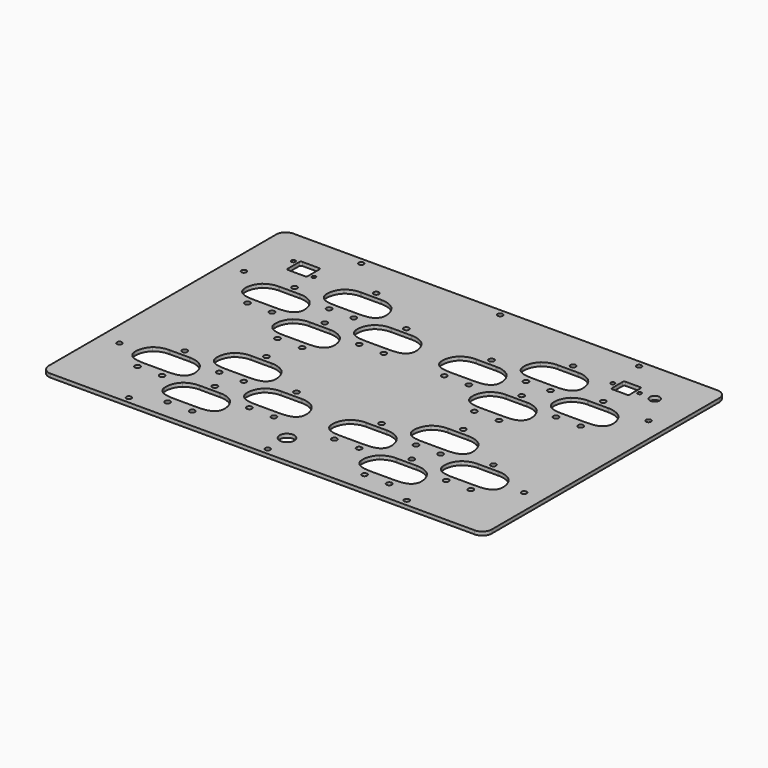
from build123d import *

# Parameters (mm, degrees)
F0_R     = 2.1
F0_R_2   = 2.2
F0_R_3   = 6
F0_R_4   = 1.625
F0_R_5   = 1.6
F0_R_6   = 4.05
F1_DEPTH = 3


# Not quite as in the source:
# - the dataset's text gives a spline's control points without its knots; the knots are read off the source's solid


with BuildPart() as f1:
    # F0 (on Top) → F1 (new body)
    with BuildSketch(Plane.XY):
        with BuildLine():
            Line((174.5, 124.8), (-174.5, 124.8))
            ThreePointArc((-174.5, 124.8), (-180.0154328933, 122.5154328933), (-182.3, 117))
            Line((-182.3, 117), (-182.3, -117))
            ThreePointArc((-182.3, -117), (-180.0154328933, -122.5154328933), (-174.5, -124.8))
            Line((-174.5, -124.8), (174.5, -124.8))
            ThreePointArc((174.5, -124.8), (180.0154328933, -122.5154328933), (182.3, -117))
            Line((182.3, -117), (182.3, 117))
            ThreePointArc((182.3, 117), (180.0154328933, 122.5154328933), (174.5, 124.8))
        make_face()
        with Locations((-114.33, -119.5)):
            Circle(F0_R, mode=Mode.SUBTRACT)
        with Locations((-137.12, -82.102)):
            Circle(F0_R_2, mode=Mode.SUBTRACT)
        with Locations((-166.5, -64)):
            Circle(F0_R, mode=Mode.SUBTRACT)
        with Locations((-116.88, -82.102)):
            Circle(F0_R_2, mode=Mode.SUBTRACT)
        with BuildLine():
            Line((-135.6612948233, -51.451130735), (-135.115026498, -51.4620000001))
            Line((-135.115026498, -51.4620000001), (-118.8944121234, -51.4620000001))
            Line((-118.8944121234, -51.4620000001), (-118.3330315352, -51.4511211146))
            ThreePointArc((-118.3330315352, -51.4511211146), (-112.5954929046, -52.4136608229), (-107.487280821, -55.1979024679))
            ThreePointArc((-107.487280821, -55.1979024679), (-103.7289593809, -60.9649156398), (-102.7756384695, -67.7821438311))
            add(Edge.make_bspline(
                [(-102.7756384695, -67.7821438311), (-102.8317808557, -68.4791518436), (-103.1342622315, -69.8522558093), (-104.1227442667, -71.7376713061), (-105.3617732771, -73.0712234734), (-106.5853971676, -73.93803931), (-107.9464485907, -74.6539246569), (-109.8851336202, -75.2963766675), (-112.5588382079, -75.7473994177), (-115.5566427484, -75.9552688032), (-117.7556974045, -75.97825395), (-118.9009345935, -75.9720000001)],
                knots=[0, 0, 0, 0, 0.125, 0.25, 0.375, 0.4375, 0.5, 0.625, 0.75, 0.875, 0.9999501857, 0.9999501857, 0.9999501857, 0.9999501857], degree=3))
            Line((-118.9009345935, -75.9720000001), (-135.1072635354, -75.9720000001))
            Line((-135.1072635354, -75.9720000001), (-135.1086333173, -75.9720000001))
            add(Edge.make_bspline(
                [(-151.2339294072, -67.7821438309), (-151.177741554, -68.4797163167), (-150.8726831114, -69.8530561961), (-149.8774581613, -71.7367332364), (-148.6340002387, -73.0683891085), (-147.4094063644, -73.9344572306), (-146.0489657757, -74.6503376548), (-144.1131861346, -75.2935631846), (-141.4445788782, -75.7458922174), (-138.4515011772, -75.954911071), (-136.2539205452, -75.9782540848), (-135.1086333173, -75.9720000001)],
                knots=[0, 0, 0, 0, 0.125, 0.25, 0.375, 0.4375, 0.5, 0.625, 0.75, 0.875, 0.9999501867, 0.9999501867, 0.9999501867, 0.9999501867], degree=3))
            ThreePointArc((-151.2339294072, -67.7821438309), (-150.2806084958, -60.9649156397), (-146.5222870557, -55.1979024678))
            ThreePointArc((-146.5222870557, -55.1979024678), (-141.4068713777, -52.411174013), (-135.6612948233, -51.451130735))
        make_face(mode=Mode.SUBTRACT)
        with Locations((-91.12, -108.602)):
            Circle(F0_R_2, mode=Mode.SUBTRACT)
        with Locations((-70.88, -108.602)):
            Circle(F0_R_2, mode=Mode.SUBTRACT)
        with BuildLine():
            Line((-89.6612948233, -77.951130735), (-89.115026498, -77.9620000001))
            Line((-89.115026498, -77.9620000001), (-72.8944121234, -77.9620000001))
            Line((-72.8944121234, -77.9620000001), (-72.3330315352, -77.9511211146))
            ThreePointArc((-72.3330315352, -77.9511211146), (-66.5954929046, -78.9136608229), (-61.487280821, -81.6979024679))
            ThreePointArc((-61.487280821, -81.6979024679), (-57.7289593809, -87.4649156398), (-56.7756384695, -94.2821438311))
            add(Edge.make_bspline(
                [(-56.7756384695, -94.2821438311), (-56.8318288861, -94.9783630519), (-57.1341419789, -96.3506841544), (-58.1219861034, -98.2355446893), (-59.3608225377, -99.5692757568), (-60.5843212484, -100.4362682741), (-61.9452692843, -101.1523501476), (-63.8838615244, -101.7950820951), (-66.5575009571, -102.2464909201), (-69.5556737218, -102.4548208566), (-71.7552033004, -102.4781051534), (-72.9009345935, -102.4720000001)],
                knots=[0.0001387542, 0.0001387542, 0.0001387542, 0.0001387542, 0.125, 0.25, 0.375, 0.4375, 0.5, 0.625, 0.75, 0.875, 1, 1, 1, 1], degree=3))
            Line((-72.9009345935, -102.4720000001), (-89.1072635354, -102.4720000001))
            Line((-89.1072635354, -102.4720000001), (-89.1086333173, -102.4720000001))
            add(Edge.make_bspline(
                [(-105.2339294072, -94.2821438309), (-105.177741554, -94.9797163167), (-104.8726831114, -96.3530561961), (-103.8774581613, -98.2367332364), (-102.6340002387, -99.5683891085), (-101.4094063644, -100.4344572306), (-100.0489657757, -101.1503376548), (-98.1131861346, -101.7935631846), (-95.4445788782, -102.2458922174), (-92.4515011772, -102.454911071), (-90.2539205452, -102.4782540848), (-89.1086333173, -102.4720000001)],
                knots=[0, 0, 0, 0, 0.125, 0.25, 0.375, 0.4375, 0.5, 0.625, 0.75, 0.875, 0.9999501867, 0.9999501867, 0.9999501867, 0.9999501867], degree=3))
            ThreePointArc((-105.2339294072, -94.2821438309), (-104.2806084958, -87.4649156397), (-100.5222870557, -81.6979024678))
            ThreePointArc((-100.5222870557, -81.6979024678), (-95.4068713777, -78.911174013), (-89.6612948233, -77.951130735))
        make_face(mode=Mode.SUBTRACT)
        with Locations((-81, -72.692)):
            Circle(F0_R_2, mode=Mode.SUBTRACT)
        with Locations((-45.12, -82.102)):
            Circle(F0_R_2, mode=Mode.SUBTRACT)
        with Locations((-24.88, -82.102)):
            Circle(F0_R_2, mode=Mode.SUBTRACT)
        with BuildLine():
            Line((-43.6612948233, -51.451130735), (-43.115026498, -51.4620000001))
            Line((-43.115026498, -51.4620000001), (-26.8944121234, -51.4620000001))
            Line((-26.8944121234, -51.4620000001), (-26.3330315352, -51.4511211146))
            ThreePointArc((-26.3330315352, -51.4511211146), (-20.5954929046, -52.4136608229), (-15.487280821, -55.1979024679))
            ThreePointArc((-15.487280821, -55.1979024679), (-11.7289593809, -60.9649156398), (-10.7756384695, -67.7821438311))
            add(Edge.make_bspline(
                [(-10.7756384695, -67.7821438311), (-10.8317808557, -68.4791518436), (-11.1342622315, -69.8522558093), (-12.1227442667, -71.7376713061), (-13.3617732771, -73.0712234734), (-14.5853971676, -73.93803931), (-15.9464485907, -74.6539246569), (-17.8851336202, -75.2963766675), (-20.5588382079, -75.7473994177), (-23.5566427484, -75.9552688032), (-25.7556974045, -75.97825395), (-26.9009345935, -75.9720000001)],
                knots=[0, 0, 0, 0, 0.125, 0.25, 0.375, 0.4375, 0.5, 0.625, 0.75, 0.875, 0.9999501857, 0.9999501857, 0.9999501857, 0.9999501857], degree=3))
            Line((-26.9009345935, -75.9720000001), (-43.1072635354, -75.9720000001))
            Line((-43.1072635354, -75.9720000001), (-43.1086333173, -75.9720000001))
            add(Edge.make_bspline(
                [(-59.2339294072, -67.7821438309), (-59.177741554, -68.4797163167), (-58.8726831114, -69.8530561961), (-57.8774581613, -71.7367332364), (-56.6340002387, -73.0683891085), (-55.4094063644, -73.9344572306), (-54.0489657757, -74.6503376548), (-52.1131861346, -75.2935631846), (-49.4445788782, -75.7458922174), (-46.4515011772, -75.954911071), (-44.2539205452, -75.9782540848), (-43.1086333173, -75.9720000001)],
                knots=[0, 0, 0, 0, 0.125, 0.25, 0.375, 0.4375, 0.5, 0.625, 0.75, 0.875, 0.9999501867, 0.9999501867, 0.9999501867, 0.9999501867], degree=3))
            ThreePointArc((-59.2339294072, -67.7821438309), (-58.2806084958, -60.9649156397), (-54.5222870557, -55.1979024678))
            ThreePointArc((-54.5222870557, -55.1979024678), (-49.4068713777, -52.411174013), (-43.6612948233, -51.451130735))
        make_face(mode=Mode.SUBTRACT)
        with Locations((-127, -46.192)):
            Circle(F0_R_2, mode=Mode.SUBTRACT)
        with Locations((-91.12, -55.602)):
            Circle(F0_R_2, mode=Mode.SUBTRACT)
        with Locations((-70.88, -55.602)):
            Circle(F0_R_2, mode=Mode.SUBTRACT)
        with BuildLine():
            Line((-89.6612948233, -24.951130735), (-89.115026498, -24.9620000001))
            Line((-89.115026498, -24.9620000001), (-72.8944121234, -24.9620000001))
            Line((-72.8944121234, -24.9620000001), (-72.3330315352, -24.9511211146))
            ThreePointArc((-72.3330315352, -24.9511211146), (-66.5954929046, -25.9136608229), (-61.487280821, -28.6979024679))
            ThreePointArc((-61.487280821, -28.6979024679), (-57.7289593809, -34.4649156398), (-56.7756384695, -41.2821438311))
            add(Edge.make_bspline(
                [(-56.7756384695, -41.2821438311), (-56.8317808557, -41.9791518436), (-57.1342622315, -43.3522558093), (-58.1227442667, -45.2376713061), (-59.3617732771, -46.5712234734), (-60.5853971676, -47.43803931), (-61.9464485907, -48.1539246569), (-63.8851336202, -48.7963766675), (-66.5588382079, -49.2473994177), (-69.5566427484, -49.4552688032), (-71.7556974045, -49.47825395), (-72.9009345935, -49.4720000001)],
                knots=[0, 0, 0, 0, 0.125, 0.25, 0.375, 0.4375, 0.5, 0.625, 0.75, 0.875, 0.9999501857, 0.9999501857, 0.9999501857, 0.9999501857], degree=3))
            Line((-72.9009345935, -49.4720000001), (-89.1072635354, -49.4720000001))
            Line((-89.1072635354, -49.4720000001), (-89.1086333173, -49.4720000001))
            add(Edge.make_bspline(
                [(-105.2339294072, -41.2821438309), (-105.177741554, -41.9797163167), (-104.8726831114, -43.3530561961), (-103.8774581613, -45.2367332364), (-102.6340002387, -46.5683891085), (-101.4094063644, -47.4344572306), (-100.0489657757, -48.1503376548), (-98.1131861346, -48.7935631846), (-95.4445788782, -49.2458922174), (-92.4515011772, -49.454911071), (-90.2539205452, -49.4782540848), (-89.1086333173, -49.4720000001)],
                knots=[0, 0, 0, 0, 0.125, 0.25, 0.375, 0.4375, 0.5, 0.625, 0.75, 0.875, 0.9999501867, 0.9999501867, 0.9999501867, 0.9999501867], degree=3))
            ThreePointArc((-105.2339294072, -41.2821438309), (-104.2806084958, -34.4649156397), (-100.5222870557, -28.6979024678))
            ThreePointArc((-100.5222870557, -28.6979024678), (-95.4068713777, -25.911174013), (-89.6612948233, -24.951130735))
        make_face(mode=Mode.SUBTRACT)
        with Locations((-35, -46.192)):
            Circle(F0_R_2, mode=Mode.SUBTRACT)
        with Locations((-81, -19.692)):
            Circle(F0_R_2, mode=Mode.SUBTRACT)
        with Locations((0, -119.5)):
            Circle(F0_R, mode=Mode.SUBTRACT)
        with Locations((0, -99.8)):
            Circle(F0_R_3, mode=Mode.SUBTRACT)
        with Locations((70.88, -108.602)):
            Circle(F0_R_2, mode=Mode.SUBTRACT)
        with Locations((91.12, -108.602)):
            Circle(F0_R_2, mode=Mode.SUBTRACT)
        with Locations((24.88, -82.102)):
            Circle(F0_R_2, mode=Mode.SUBTRACT)
        with Locations((45.12, -82.102)):
            Circle(F0_R_2, mode=Mode.SUBTRACT)
        with BuildLine():
            Line((26.3387051767, -51.451130735), (26.884973502, -51.4620000001))
            Line((26.884973502, -51.4620000001), (43.1055878766, -51.4620000001))
            Line((43.1055878766, -51.4620000001), (43.6669684648, -51.4511211146))
            ThreePointArc((43.6669684648, -51.4511211146), (49.4045070954, -52.4136608229), (54.512719179, -55.1979024679))
            ThreePointArc((54.512719179, -55.1979024679), (58.2710406191, -60.9649156398), (59.2243615305, -67.7821438311))
            add(Edge.make_bspline(
                [(59.2243615305, -67.7821438311), (59.1682191443, -68.4791518436), (58.8657377685, -69.8522558093), (57.8772557333, -71.7376713061), (56.6382267229, -73.0712234734), (55.4146028324, -73.93803931), (54.0535514093, -74.6539246569), (52.1148663798, -75.2963766675), (49.4411617921, -75.7473994177), (46.4433572516, -75.9552688032), (44.2443025955, -75.97825395), (43.0990654065, -75.9720000001)],
                knots=[0, 0, 0, 0, 0.125, 0.25, 0.375, 0.4375, 0.5, 0.625, 0.75, 0.875, 0.9999501857, 0.9999501857, 0.9999501857, 0.9999501857], degree=3))
            Line((43.0990654065, -75.9720000001), (26.8927364646, -75.9720000001))
            Line((26.8927364646, -75.9720000001), (26.8913666827, -75.9720000001))
            add(Edge.make_bspline(
                [(10.7660705928, -67.7821438309), (10.822258446, -68.4797163167), (11.1273168886, -69.8530561961), (12.1225418387, -71.7367332364), (13.3659997613, -73.0683891085), (14.5905936356, -73.9344572306), (15.9510342243, -74.6503376548), (17.8868138654, -75.2935631846), (20.5554211218, -75.7458922174), (23.5484988228, -75.954911071), (25.7460794548, -75.9782540848), (26.8913666827, -75.9720000001)],
                knots=[0, 0, 0, 0, 0.125, 0.25, 0.375, 0.4375, 0.5, 0.625, 0.75, 0.875, 0.9999501867, 0.9999501867, 0.9999501867, 0.9999501867], degree=3))
            ThreePointArc((10.7660705928, -67.7821438309), (11.7193915042, -60.9649156397), (15.4777129443, -55.1979024678))
            ThreePointArc((15.4777129443, -55.1979024678), (20.5931286223, -52.411174013), (26.3387051767, -51.451130735))
        make_face(mode=Mode.SUBTRACT)
        with BuildLine():
            Line((72.3387051767, -77.951130735), (72.884973502, -77.9620000001))
            Line((72.884973502, -77.9620000001), (89.1055878766, -77.9620000001))
            Line((89.1055878766, -77.9620000001), (89.6669684648, -77.9511211146))
            ThreePointArc((89.6669684648, -77.9511211146), (95.4045070954, -78.9136608229), (100.512719179, -81.6979024679))
            ThreePointArc((100.512719179, -81.6979024679), (104.2710406191, -87.4649156398), (105.2243615305, -94.2821438311))
            add(Edge.make_bspline(
                [(105.2243615305, -94.2821438311), (105.1682191443, -94.9791518436), (104.8657377685, -96.3522558093), (103.8772557333, -98.2376713061), (102.6382267229, -99.5712234734), (101.4146028324, -100.43803931), (100.0535514093, -101.1539246569), (98.1148663798, -101.7963766675), (95.4411617921, -102.2473994177), (92.4433572516, -102.4552688032), (90.2443025955, -102.47825395), (89.0990654065, -102.4720000001)],
                knots=[0, 0, 0, 0, 0.125, 0.25, 0.375, 0.4375, 0.5, 0.625, 0.75, 0.875, 0.9999501857, 0.9999501857, 0.9999501857, 0.9999501857], degree=3))
            Line((89.0990654065, -102.4720000001), (72.8927364646, -102.4720000001))
            Line((72.8927364646, -102.4720000001), (72.8913666827, -102.4720000001))
            add(Edge.make_bspline(
                [(56.7660705928, -94.2821438309), (56.822258446, -94.9797163167), (57.1273168886, -96.3530561961), (58.1225418387, -98.2367332364), (59.3659997613, -99.5683891085), (60.5905936356, -100.4344572306), (61.9510342243, -101.1503376548), (63.8868138654, -101.7935631846), (66.5554211218, -102.2458922174), (69.5484988228, -102.454911071), (71.7460794548, -102.4782540848), (72.8913666827, -102.4720000001)],
                knots=[0, 0, 0, 0, 0.125, 0.25, 0.375, 0.4375, 0.5, 0.625, 0.75, 0.875, 0.9999501867, 0.9999501867, 0.9999501867, 0.9999501867], degree=3))
            ThreePointArc((56.7660705928, -94.2821438309), (57.7193915042, -87.4649156397), (61.4777129443, -81.6979024678))
            ThreePointArc((61.4777129443, -81.6979024678), (66.5931286223, -78.911174013), (72.3387051767, -77.951130735))
        make_face(mode=Mode.SUBTRACT)
        with Locations((81, -72.692)):
            Circle(F0_R_2, mode=Mode.SUBTRACT)
        with Locations((114.33, -119.5)):
            Circle(F0_R, mode=Mode.SUBTRACT)
        with Locations((116.88, -82.102)):
            Circle(F0_R_2, mode=Mode.SUBTRACT)
        with BuildLine():
            Line((118.3387051767, -51.451130735), (118.884973502, -51.4620000001))
            Line((118.884973502, -51.4620000001), (135.1055878766, -51.4620000001))
            Line((135.1055878766, -51.4620000001), (135.6669684648, -51.4511211146))
            ThreePointArc((135.6669684648, -51.4511211146), (141.4045070954, -52.4136608229), (146.512719179, -55.1979024679))
            ThreePointArc((146.512719179, -55.1979024679), (150.2710406191, -60.9649156398), (151.2243615305, -67.7821438311))
            add(Edge.make_bspline(
                [(151.2243615305, -67.7821438311), (151.1682191443, -68.4791518436), (150.8657377685, -69.8522558093), (149.8772557333, -71.7376713061), (148.6382267229, -73.0712234734), (147.4146028324, -73.93803931), (146.0535514093, -74.6539246569), (144.1148663798, -75.2963766675), (141.4411617921, -75.7473994177), (138.4433572516, -75.9552688032), (136.2443025955, -75.97825395), (135.0990654065, -75.9720000001)],
                knots=[0, 0, 0, 0, 0.125, 0.25, 0.375, 0.4375, 0.5, 0.625, 0.75, 0.875, 0.9999501857, 0.9999501857, 0.9999501857, 0.9999501857], degree=3))
            Line((135.0990654065, -75.9720000001), (118.8927364646, -75.9720000001))
            Line((118.8927364646, -75.9720000001), (118.8913666827, -75.9720000001))
            add(Edge.make_bspline(
                [(102.7660705928, -67.7821438309), (102.822258446, -68.4797163167), (103.1273168886, -69.8530561961), (104.1225418387, -71.7367332364), (105.3659997613, -73.0683891085), (106.5905936356, -73.9344572306), (107.9510342243, -74.6503376548), (109.8868138654, -75.2935631846), (112.5554211218, -75.7458922174), (115.5484988228, -75.954911071), (117.7460794548, -75.9782540848), (118.8913666827, -75.9720000001)],
                knots=[0, 0, 0, 0, 0.125, 0.25, 0.375, 0.4375, 0.5, 0.625, 0.75, 0.875, 0.9999501867, 0.9999501867, 0.9999501867, 0.9999501867], degree=3))
            ThreePointArc((102.7660705928, -67.7821438309), (103.7193915042, -60.9649156397), (107.4777129443, -55.1979024678))
            ThreePointArc((107.4777129443, -55.1979024678), (112.5931286223, -52.411174013), (118.3387051767, -51.451130735))
        make_face(mode=Mode.SUBTRACT)
        with Locations((137.12, -82.102)):
            Circle(F0_R_2, mode=Mode.SUBTRACT)
        with Locations((166.5, -64)):
            Circle(F0_R, mode=Mode.SUBTRACT)
        with Locations((35, -46.192)):
            Circle(F0_R_2, mode=Mode.SUBTRACT)
        with Locations((70.88, -55.602)):
            Circle(F0_R_2, mode=Mode.SUBTRACT)
        with Locations((91.12, -55.602)):
            Circle(F0_R_2, mode=Mode.SUBTRACT)
        with BuildLine():
            Line((72.3387051767, -24.951130735), (72.884973502, -24.9620000001))
            Line((72.884973502, -24.9620000001), (89.1055878766, -24.9620000001))
            Line((89.1055878766, -24.9620000001), (89.6669684648, -24.9511211146))
            ThreePointArc((89.6669684648, -24.9511211146), (95.4045070954, -25.9136608229), (100.512719179, -28.6979024679))
            ThreePointArc((100.512719179, -28.6979024679), (104.2710406191, -34.4649156398), (105.2243615305, -41.2821438311))
            add(Edge.make_bspline(
                [(105.2243615305, -41.2821438311), (105.1682191443, -41.9791518436), (104.8657377685, -43.3522558093), (103.8772557333, -45.2376713061), (102.6382267229, -46.5712234734), (101.4146028324, -47.43803931), (100.0535514093, -48.1539246569), (98.1148663798, -48.7963766675), (95.4411617921, -49.2473994177), (92.4433572516, -49.4552688032), (90.2443025955, -49.47825395), (89.0990654065, -49.4720000001)],
                knots=[0, 0, 0, 0, 0.125, 0.25, 0.375, 0.4375, 0.5, 0.625, 0.75, 0.875, 0.9999501857, 0.9999501857, 0.9999501857, 0.9999501857], degree=3))
            Line((89.0990654065, -49.4720000001), (72.8927364646, -49.4720000001))
            Line((72.8927364646, -49.4720000001), (72.8913666827, -49.4720000001))
            add(Edge.make_bspline(
                [(56.7660705928, -41.2821438309), (56.822258446, -41.9797163167), (57.1273168886, -43.3530561961), (58.1225418387, -45.2367332364), (59.3659997613, -46.5683891085), (60.5905936356, -47.4344572306), (61.9510342243, -48.1503376548), (63.8868138654, -48.7935631846), (66.5554211218, -49.2458922174), (69.5484988228, -49.454911071), (71.7460794548, -49.4782540848), (72.8913666827, -49.4720000001)],
                knots=[0, 0, 0, 0, 0.125, 0.25, 0.375, 0.4375, 0.5, 0.625, 0.75, 0.875, 0.9999501867, 0.9999501867, 0.9999501867, 0.9999501867], degree=3))
            ThreePointArc((56.7660705928, -41.2821438309), (57.7193915042, -34.4649156397), (61.4777129443, -28.6979024678))
            ThreePointArc((61.4777129443, -28.6979024678), (66.5931286223, -25.911174013), (72.3387051767, -24.951130735))
        make_face(mode=Mode.SUBTRACT)
        with Locations((81, -19.692)):
            Circle(F0_R_2, mode=Mode.SUBTRACT)
        with Locations((127, -46.192)):
            Circle(F0_R_2, mode=Mode.SUBTRACT)
        with Locations((-137.12, 30.898)):
            Circle(F0_R_2, mode=Mode.SUBTRACT)
        with Locations((-116.88, 30.898)):
            Circle(F0_R_2, mode=Mode.SUBTRACT)
        with BuildLine():
            Line((-135.6612948233, 61.548869265), (-135.115026498, 61.5379999999))
            Line((-135.115026498, 61.5379999999), (-118.8944121234, 61.5379999999))
            Line((-118.8944121234, 61.5379999999), (-118.3330315352, 61.5488788854))
            ThreePointArc((-118.3330315352, 61.5488788854), (-112.5954929046, 60.5863391771), (-107.487280821, 57.8020975321))
            ThreePointArc((-107.487280821, 57.8020975321), (-103.7289593809, 52.0350843602), (-102.7756384695, 45.2178561689))
            add(Edge.make_bspline(
                [(-102.7756384695, 45.2178561689), (-102.8317808557, 44.5208481564), (-103.1342622315, 43.1477441907), (-104.1227442667, 41.2623286939), (-105.3617732771, 39.9287765266), (-106.5853971676, 39.06196069), (-107.9464485907, 38.3460753431), (-109.8851336202, 37.7036233325), (-112.5588382079, 37.2526005823), (-115.5566427484, 37.0447311968), (-117.7556974045, 37.02174605), (-118.9009345935, 37.0279999999)],
                knots=[0, 0, 0, 0, 0.125, 0.25, 0.375, 0.4375, 0.5, 0.625, 0.75, 0.875, 0.9999501857, 0.9999501857, 0.9999501857, 0.9999501857], degree=3))
            Line((-118.9009345935, 37.0279999999), (-135.1072635354, 37.0279999999))
            Line((-135.1072635354, 37.0279999999), (-135.1086333173, 37.0279999999))
            add(Edge.make_bspline(
                [(-151.2339294072, 45.2178561691), (-151.177741554, 44.5202836833), (-150.8726831114, 43.1469438039), (-149.8774581613, 41.2632667636), (-148.6340002387, 39.9316108915), (-147.4094063644, 39.0655427694), (-146.0489657757, 38.3496623452), (-144.1131861346, 37.7064368154), (-141.4445788782, 37.2541077826), (-138.4515011772, 37.045088929), (-136.2539205452, 37.0217459152), (-135.1086333173, 37.0279999999)],
                knots=[0, 0, 0, 0, 0.125, 0.25, 0.375, 0.4375, 0.5, 0.625, 0.75, 0.875, 0.9999501867, 0.9999501867, 0.9999501867, 0.9999501867], degree=3))
            ThreePointArc((-151.2339294072, 45.2178561691), (-150.2806084958, 52.0350843603), (-146.5222870557, 57.8020975322))
            ThreePointArc((-146.5222870557, 57.8020975322), (-141.4068713777, 60.588825987), (-135.6612948233, 61.548869265))
        make_face(mode=Mode.SUBTRACT)
        with Locations((-91.12, 4.398)):
            Circle(F0_R_2, mode=Mode.SUBTRACT)
        with Locations((-70.88, 4.398)):
            Circle(F0_R_2, mode=Mode.SUBTRACT)
        with BuildLine():
            Line((-89.6612948233, 35.048869265), (-89.115026498, 35.0379999999))
            Line((-89.115026498, 35.0379999999), (-72.8944121234, 35.0379999999))
            Line((-72.8944121234, 35.0379999999), (-72.3330315352, 35.0488788854))
            ThreePointArc((-72.3330315352, 35.0488788854), (-66.5954929046, 34.0863391771), (-61.487280821, 31.3020975321))
            ThreePointArc((-61.487280821, 31.3020975321), (-57.7289593809, 25.5350843602), (-56.7756384695, 18.7178561689))
            add(Edge.make_bspline(
                [(-56.7756384695, 18.7178561689), (-56.8317808557, 18.0208481564), (-57.1342622315, 16.6477441907), (-58.1227442667, 14.7623286939), (-59.3617732771, 13.4287765266), (-60.5853971676, 12.56196069), (-61.9464485907, 11.8460753431), (-63.8851336202, 11.2036233325), (-66.5588382079, 10.7526005823), (-69.5566427484, 10.5447311968), (-71.7556974045, 10.52174605), (-72.9009345935, 10.5279999999)],
                knots=[0, 0, 0, 0, 0.125, 0.25, 0.375, 0.4375, 0.5, 0.625, 0.75, 0.875, 0.9999501857, 0.9999501857, 0.9999501857, 0.9999501857], degree=3))
            Line((-72.9009345935, 10.5279999999), (-89.1072635354, 10.5279999999))
            Line((-89.1072635354, 10.5279999999), (-89.1086333173, 10.5279999999))
            add(Edge.make_bspline(
                [(-105.2339294072, 18.7178561691), (-105.177741554, 18.0202836833), (-104.8726831114, 16.6469438039), (-103.8774581613, 14.7632667636), (-102.6340002387, 13.4316108915), (-101.4094063644, 12.5655427694), (-100.0489657757, 11.8496623452), (-98.1131861346, 11.2064368154), (-95.4445788782, 10.7541077826), (-92.4515011772, 10.545088929), (-90.2539205452, 10.5217459152), (-89.1086333173, 10.5279999999)],
                knots=[0, 0, 0, 0, 0.125, 0.25, 0.375, 0.4375, 0.5, 0.625, 0.75, 0.875, 0.9999501867, 0.9999501867, 0.9999501867, 0.9999501867], degree=3))
            ThreePointArc((-105.2339294072, 18.7178561691), (-104.2806084958, 25.5350843603), (-100.5222870557, 31.3020975322))
            ThreePointArc((-100.5222870557, 31.3020975322), (-95.4068713777, 34.088825987), (-89.6612948233, 35.048869265))
        make_face(mode=Mode.SUBTRACT)
        with Locations((-45.12, 30.898)):
            Circle(F0_R_2, mode=Mode.SUBTRACT)
        with Locations((-24.88, 30.898)):
            Circle(F0_R_2, mode=Mode.SUBTRACT)
        with Locations((-81, 40.308)):
            Circle(F0_R_2, mode=Mode.SUBTRACT)
        with Locations((-91.12, 57.398)):
            Circle(F0_R_2, mode=Mode.SUBTRACT)
        with Locations((-70.88, 57.398)):
            Circle(F0_R_2, mode=Mode.SUBTRACT)
        with BuildLine():
            Line((-43.6612948233, 61.548869265), (-43.115026498, 61.5379999999))
            Line((-43.115026498, 61.5379999999), (-26.8944121234, 61.5379999999))
            Line((-26.8944121234, 61.5379999999), (-26.3330315352, 61.5488788854))
            ThreePointArc((-26.3330315352, 61.5488788854), (-20.5954929046, 60.5863391771), (-15.487280821, 57.8020975321))
            ThreePointArc((-15.487280821, 57.8020975321), (-11.7282191214, 52.0352577574), (-10.7742686876, 45.2178561689))
            add(Edge.make_bspline(
                [(-10.7742686876, 45.2178561689), (-10.8304110738, 44.5208481564), (-11.1328924496, 43.1477441907), (-12.1213744847, 41.2623286939), (-13.3604034952, 39.9287765266), (-14.5840273857, 39.06196069), (-15.9450788087, 38.3460753431), (-17.8837638383, 37.7036233325), (-20.557468426, 37.2526005823), (-23.5552729664, 37.0447311968), (-25.7543276226, 37.02174605), (-26.8995648116, 37.0279999999)],
                knots=[0, 0, 0, 0, 0.125, 0.25, 0.375, 0.4375, 0.5, 0.625, 0.75, 0.875, 0.9999501857, 0.9999501857, 0.9999501857, 0.9999501857], degree=3))
            Line((-26.8995648116, 37.0279999999), (-43.1072635354, 37.0279999999))
            add(Edge.make_bspline(
                [(-59.2325596253, 45.2178561691), (-59.1763212388, 44.5210734563), (-58.8714315071, 43.1485163208), (-57.876846428, 41.2653920745), (-56.633580812, 39.9335566586), (-55.4091120122, 39.0673117119), (-54.0487748122, 38.3512348451), (-52.1130880742, 37.7077297918), (-49.4445461628, 37.255015412), (-46.4511010398, 37.0455365283), (-44.2530455057, 37.0218945801), (-43.1072635354, 37.0279999999)],
                knots=[0.0001386451, 0.0001386451, 0.0001386451, 0.0001386451, 0.125, 0.25, 0.375, 0.4375, 0.5, 0.625, 0.75, 0.875, 1, 1, 1, 1], degree=3))
            ThreePointArc((-59.2325596253, 45.2178561691), (-58.2798682404, 52.0349109767), (-54.5222870557, 57.8020975322))
            ThreePointArc((-54.5222870557, 57.8020975322), (-49.4068713777, 60.588825987), (-43.6612948233, 61.548869265))
        make_face(mode=Mode.SUBTRACT)
        with Locations((-166.5, 64)):
            Circle(F0_R, mode=Mode.SUBTRACT)
        with BuildLine():
            ThreePointArc((-146.775, 96.295), (-146.370807358, 97.270807358), (-145.395, 97.675))
            Line((-145.395, 97.675), (-131.605, 97.675))
            ThreePointArc((-131.605, 97.675), (-130.629192642, 97.270807358), (-130.225, 96.295))
            Line((-130.225, 96.295), (-130.225, 84.505))
            ThreePointArc((-130.225, 84.505), (-130.629192642, 83.529192642), (-131.605, 83.125))
            Line((-131.605, 83.125), (-145.395, 83.125))
            ThreePointArc((-145.395, 83.125), (-146.370807358, 83.529192642), (-146.775, 84.505))
            Line((-146.775, 84.505), (-146.775, 96.295))
        make_face(mode=Mode.SUBTRACT)
        with Locations((-127, 66.808)):
            Circle(F0_R_2, mode=Mode.SUBTRACT)
        with Locations((-126.5, 85.9)):
            Circle(F0_R_4, mode=Mode.SUBTRACT)
        with Locations((-150.5, 94.9)):
            Circle(F0_R_4, mode=Mode.SUBTRACT)
        with Locations((-114.33, 119.5)):
            Circle(F0_R, mode=Mode.SUBTRACT)
        with BuildLine():
            Line((-89.6612948233, 88.048869265), (-89.115026498, 88.0379999999))
            Line((-89.115026498, 88.0379999999), (-72.8944121234, 88.0379999999))
            Line((-72.8944121234, 88.0379999999), (-72.3330315352, 88.0488788854))
            ThreePointArc((-72.3330315352, 88.0488788854), (-66.5954929046, 87.0863391771), (-61.487280821, 84.3020975321))
            ThreePointArc((-61.487280821, 84.3020975321), (-57.7289593809, 78.5350843602), (-56.7756384695, 71.7178561689))
            add(Edge.make_bspline(
                [(-56.7756384695, 71.7178561689), (-56.8317808557, 71.0208481564), (-57.1342622315, 69.6477441907), (-58.1227442667, 67.7623286939), (-59.3617732771, 66.4287765266), (-60.5853971676, 65.56196069), (-61.9464485907, 64.8460753431), (-63.8851336202, 64.2036233325), (-66.5588382079, 63.7526005823), (-69.5566427484, 63.5447311968), (-71.7556974045, 63.52174605), (-72.9009345935, 63.5279999999)],
                knots=[0, 0, 0, 0, 0.125, 0.25, 0.375, 0.4375, 0.5, 0.625, 0.75, 0.875, 0.9999501857, 0.9999501857, 0.9999501857, 0.9999501857], degree=3))
            Line((-72.9009345935, 63.5279999999), (-89.1072635354, 63.5279999999))
            Line((-89.1072635354, 63.5279999999), (-89.1086333173, 63.5279999999))
            add(Edge.make_bspline(
                [(-105.2339294072, 71.7178561691), (-105.177741554, 71.0202836833), (-104.8726831114, 69.6469438039), (-103.8774581613, 67.7632667636), (-102.6340002387, 66.4316108915), (-101.4094063644, 65.5655427694), (-100.0489657757, 64.8496623452), (-98.1131861346, 64.2064368154), (-95.4445788782, 63.7541077826), (-92.4515011772, 63.545088929), (-90.2539205452, 63.5217459152), (-89.1086333173, 63.5279999999)],
                knots=[0, 0, 0, 0, 0.125, 0.25, 0.375, 0.4375, 0.5, 0.625, 0.75, 0.875, 0.9999501867, 0.9999501867, 0.9999501867, 0.9999501867], degree=3))
            ThreePointArc((-105.2339294072, 71.7178561691), (-104.2806084958, 78.5350843603), (-100.5222870557, 84.3020975322))
            ThreePointArc((-100.5222870557, 84.3020975322), (-95.4068713777, 87.088825987), (-89.6612948233, 88.048869265))
        make_face(mode=Mode.SUBTRACT)
        with Locations((-81, 93.308)):
            Circle(F0_R_2, mode=Mode.SUBTRACT)
        with Locations((-35, 66.808)):
            Circle(F0_R_2, mode=Mode.SUBTRACT)
        with Locations((24.88, 30.898)):
            Circle(F0_R_2, mode=Mode.SUBTRACT)
        with Locations((45.12, 30.898)):
            Circle(F0_R_2, mode=Mode.SUBTRACT)
        with Locations((70.88, 4.398)):
            Circle(F0_R_2, mode=Mode.SUBTRACT)
        with Locations((91.12, 4.398)):
            Circle(F0_R_2, mode=Mode.SUBTRACT)
        with BuildLine():
            Line((72.3387051767, 35.048869265), (72.884973502, 35.0379999999))
            Line((72.884973502, 35.0379999999), (89.1055878766, 35.0379999999))
            Line((89.1055878766, 35.0379999999), (89.6669684648, 35.0488788854))
            ThreePointArc((89.6669684648, 35.0488788854), (95.4045070954, 34.0863391771), (100.512719179, 31.3020975321))
            ThreePointArc((100.512719179, 31.3020975321), (104.2710406191, 25.5350843602), (105.2243615305, 18.7178561689))
            add(Edge.make_bspline(
                [(105.2243615305, 18.7178561689), (105.1681711139, 18.0216369481), (104.8658580211, 16.6493158456), (103.8780138966, 14.7644553107), (102.6391774623, 13.4307242432), (101.4156787516, 12.5637317259), (100.0547307157, 11.8476498524), (98.1161384756, 11.2049179049), (95.4424990429, 10.7535090799), (92.4443262782, 10.5451791434), (90.2447966996, 10.5218948466), (89.0990654065, 10.5279999999)],
                knots=[0.0001387542, 0.0001387542, 0.0001387542, 0.0001387542, 0.125, 0.25, 0.375, 0.4375, 0.5, 0.625, 0.75, 0.875, 1, 1, 1, 1], degree=3))
            Line((89.0990654065, 10.5279999999), (72.8927364646, 10.5279999999))
            Line((72.8927364646, 10.5279999999), (72.8913666827, 10.5279999999))
            add(Edge.make_bspline(
                [(56.7660705928, 18.7178561691), (56.822258446, 18.0202836833), (57.1273168886, 16.6469438039), (58.1225418387, 14.7632667636), (59.3659997613, 13.4316108915), (60.5905936356, 12.5655427694), (61.9510342243, 11.8496623452), (63.8868138654, 11.2064368154), (66.5554211218, 10.7541077826), (69.5484988228, 10.545088929), (71.7460794548, 10.5217459152), (72.8913666827, 10.5279999999)],
                knots=[0, 0, 0, 0, 0.125, 0.25, 0.375, 0.4375, 0.5, 0.625, 0.75, 0.875, 0.9999501867, 0.9999501867, 0.9999501867, 0.9999501867], degree=3))
            ThreePointArc((56.7660705928, 18.7178561691), (57.7193915042, 25.5350843603), (61.4777129443, 31.3020975322))
            ThreePointArc((61.4777129443, 31.3020975322), (66.5931286223, 34.088825987), (72.3387051767, 35.048869265))
        make_face(mode=Mode.SUBTRACT)
        with BuildLine():
            Line((26.3387051767, 61.548869265), (26.884973502, 61.5379999999))
            Line((26.884973502, 61.5379999999), (43.1055878766, 61.5379999999))
            Line((43.1055878766, 61.5379999999), (43.6669684648, 61.5488788854))
            ThreePointArc((43.6669684648, 61.5488788854), (49.4045070954, 60.5863391771), (54.512719179, 57.8020975321))
            ThreePointArc((54.512719179, 57.8020975321), (58.2710406191, 52.0350843602), (59.2243615305, 45.2178561689))
            add(Edge.make_bspline(
                [(59.2243615305, 45.2178561689), (59.1681711139, 44.5216369481), (58.8658580211, 43.1493158456), (57.8780138966, 41.2644553107), (56.6391774623, 39.9307242432), (55.4156787516, 39.0637317259), (54.0547307157, 38.3476498524), (52.1161384756, 37.7049179049), (49.4424990429, 37.2535090799), (46.4443262782, 37.0451791434), (44.2447966996, 37.0218948466), (43.0990654065, 37.0279999999)],
                knots=[0.0001387542, 0.0001387542, 0.0001387542, 0.0001387542, 0.125, 0.25, 0.375, 0.4375, 0.5, 0.625, 0.75, 0.875, 1, 1, 1, 1], degree=3))
            Line((43.0990654065, 37.0279999999), (26.8927364646, 37.0279999999))
            Line((26.8927364646, 37.0279999999), (26.8913666827, 37.0279999999))
            add(Edge.make_bspline(
                [(10.7660705928, 45.2178561691), (10.822258446, 44.5202836833), (11.1273168886, 43.1469438039), (12.1225418387, 41.2632667636), (13.3659997613, 39.9316108915), (14.5905936356, 39.0655427694), (15.9510342243, 38.3496623452), (17.8868138654, 37.7064368154), (20.5554211218, 37.2541077826), (23.5484988228, 37.045088929), (25.7460794548, 37.0217459152), (26.8913666827, 37.0279999999)],
                knots=[0, 0, 0, 0, 0.125, 0.25, 0.375, 0.4375, 0.5, 0.625, 0.75, 0.875, 0.9999501867, 0.9999501867, 0.9999501867, 0.9999501867], degree=3))
            ThreePointArc((10.7660705928, 45.2178561691), (11.7193915042, 52.0350843603), (15.4777129443, 57.8020975322))
            ThreePointArc((15.4777129443, 57.8020975322), (20.5931286223, 60.588825987), (26.3387051767, 61.548869265))
        make_face(mode=Mode.SUBTRACT)
        with Locations((81, 40.308)):
            Circle(F0_R_2, mode=Mode.SUBTRACT)
        with Locations((70.88, 57.398)):
            Circle(F0_R_2, mode=Mode.SUBTRACT)
        with Locations((91.12, 57.398)):
            Circle(F0_R_2, mode=Mode.SUBTRACT)
        with Locations((116.88, 30.898)):
            Circle(F0_R_2, mode=Mode.SUBTRACT)
        with Locations((137.12, 30.898)):
            Circle(F0_R_2, mode=Mode.SUBTRACT)
        with BuildLine():
            Line((118.3387051767, 61.548869265), (118.884973502, 61.5379999999))
            Line((118.884973502, 61.5379999999), (135.1055878766, 61.5379999999))
            Line((135.1055878766, 61.5379999999), (135.6669684648, 61.5488788854))
            ThreePointArc((135.6669684648, 61.5488788854), (141.4045070954, 60.5863391771), (146.512719179, 57.8020975321))
            ThreePointArc((146.512719179, 57.8020975321), (150.2710406191, 52.0350843602), (151.2243615305, 45.2178561689))
            add(Edge.make_bspline(
                [(151.2243615305, 45.2178561689), (151.1681711139, 44.5216369481), (150.8658580211, 43.1493158456), (149.8780138966, 41.2644553107), (148.6391774623, 39.9307242432), (147.4156787516, 39.0637317259), (146.0547307157, 38.3476498524), (144.1161384756, 37.7049179049), (141.4424990429, 37.2535090799), (138.4443262782, 37.0451791434), (136.2447966996, 37.0218948466), (135.0990654065, 37.0279999999)],
                knots=[0.0001387542, 0.0001387542, 0.0001387542, 0.0001387542, 0.125, 0.25, 0.375, 0.4375, 0.5, 0.625, 0.75, 0.875, 1, 1, 1, 1], degree=3))
            Line((135.0990654065, 37.0279999999), (118.8927364646, 37.0279999999))
            Line((118.8927364646, 37.0279999999), (118.8913666827, 37.0279999999))
            add(Edge.make_bspline(
                [(102.7660705928, 45.2178561691), (102.822258446, 44.5202836833), (103.1273168886, 43.1469438039), (104.1225418387, 41.2632667636), (105.3659997613, 39.9316108915), (106.5905936356, 39.0655427694), (107.9510342243, 38.3496623452), (109.8868138654, 37.7064368154), (112.5554211218, 37.2541077826), (115.5484988228, 37.045088929), (117.7460794548, 37.0217459152), (118.8913666827, 37.0279999999)],
                knots=[0, 0, 0, 0, 0.125, 0.25, 0.375, 0.4375, 0.5, 0.625, 0.75, 0.875, 0.9999501867, 0.9999501867, 0.9999501867, 0.9999501867], degree=3))
            ThreePointArc((102.7660705928, 45.2178561691), (103.7193915042, 52.0350843603), (107.4777129443, 57.8020975322))
            ThreePointArc((107.4777129443, 57.8020975322), (112.5931286223, 60.588825987), (118.3387051767, 61.548869265))
        make_face(mode=Mode.SUBTRACT)
        with Locations((35, 66.808)):
            Circle(F0_R_2, mode=Mode.SUBTRACT)
        with BuildLine():
            Line((72.3387051767, 88.048869265), (72.884973502, 88.0379999999))
            Line((72.884973502, 88.0379999999), (89.1055878766, 88.0379999999))
            Line((89.1055878766, 88.0379999999), (89.6669684648, 88.0488788854))
            ThreePointArc((89.6669684648, 88.0488788854), (95.4045070954, 87.0863391771), (100.512719179, 84.3020975321))
            ThreePointArc((100.512719179, 84.3020975321), (104.2710406191, 78.5350843602), (105.2243615305, 71.7178561689))
            add(Edge.make_bspline(
                [(105.2243615305, 71.7178561689), (105.1681711139, 71.0216369481), (104.8658580211, 69.6493158456), (103.8780138966, 67.7644553107), (102.6391774623, 66.4307242432), (101.4156787516, 65.5637317259), (100.0547307157, 64.8476498524), (98.1161384756, 64.2049179049), (95.4424990429, 63.7535090799), (92.4443262782, 63.5451791434), (90.2447966996, 63.5218948466), (89.0990654065, 63.5279999999)],
                knots=[0.0001387542, 0.0001387542, 0.0001387542, 0.0001387542, 0.125, 0.25, 0.375, 0.4375, 0.5, 0.625, 0.75, 0.875, 1, 1, 1, 1], degree=3))
            Line((89.0990654065, 63.5279999999), (72.8927364646, 63.5279999999))
            Line((72.8927364646, 63.5279999999), (72.8913666827, 63.5279999999))
            add(Edge.make_bspline(
                [(56.7660705928, 71.7178561691), (56.822258446, 71.0202836833), (57.1273168886, 69.6469438039), (58.1225418387, 67.7632667636), (59.3659997613, 66.4316108915), (60.5905936356, 65.5655427694), (61.9510342243, 64.8496623452), (63.8868138654, 64.2064368154), (66.5554211218, 63.7541077826), (69.5484988228, 63.545088929), (71.7460794548, 63.5217459152), (72.8913666827, 63.5279999999)],
                knots=[0, 0, 0, 0, 0.125, 0.25, 0.375, 0.4375, 0.5, 0.625, 0.75, 0.875, 0.9999501867, 0.9999501867, 0.9999501867, 0.9999501867], degree=3))
            ThreePointArc((56.7660705928, 71.7178561691), (57.7193915042, 78.5350843603), (61.4777129443, 84.3020975322))
            ThreePointArc((61.4777129443, 84.3020975322), (66.5931286223, 87.088825987), (72.3387051767, 88.048869265))
        make_face(mode=Mode.SUBTRACT)
        with Locations((81, 93.308)):
            Circle(F0_R_2, mode=Mode.SUBTRACT)
        with Locations((0, 119.5)):
            Circle(F0_R, mode=Mode.SUBTRACT)
        with Locations((127, 66.808)):
            Circle(F0_R_2, mode=Mode.SUBTRACT)
        with Locations((116, 90.4)):
            Circle(F0_R_5, mode=Mode.SUBTRACT)
        with BuildLine():
            ThreePointArc((119.725, 95.895), (120.0999033201, 96.8000966799), (121.005, 97.175))
            Line((121.005, 97.175), (132.995, 97.175))
            ThreePointArc((132.995, 97.175), (133.9000966799, 96.8000966799), (134.275, 95.895))
            Line((134.275, 95.895), (134.275, 84.905))
            ThreePointArc((134.275, 84.905), (133.9000966799, 83.9999033201), (132.995, 83.625))
            Line((132.995, 83.625), (121.005, 83.625))
            ThreePointArc((121.005, 83.625), (120.0999033201, 83.9999033201), (119.725, 84.905))
            Line((119.725, 84.905), (119.725, 95.895))
        make_face(mode=Mode.SUBTRACT)
        with Locations((166.5, 64)):
            Circle(F0_R, mode=Mode.SUBTRACT)
        with Locations((138, 90.4)):
            Circle(F0_R_5, mode=Mode.SUBTRACT)
        with Locations((150.5, 90.4)):
            Circle(F0_R_6, mode=Mode.SUBTRACT)
        with Locations((114.33, 119.5)):
            Circle(F0_R, mode=Mode.SUBTRACT)
    extrude(amount=F1_DEPTH)


solid = f1.part
